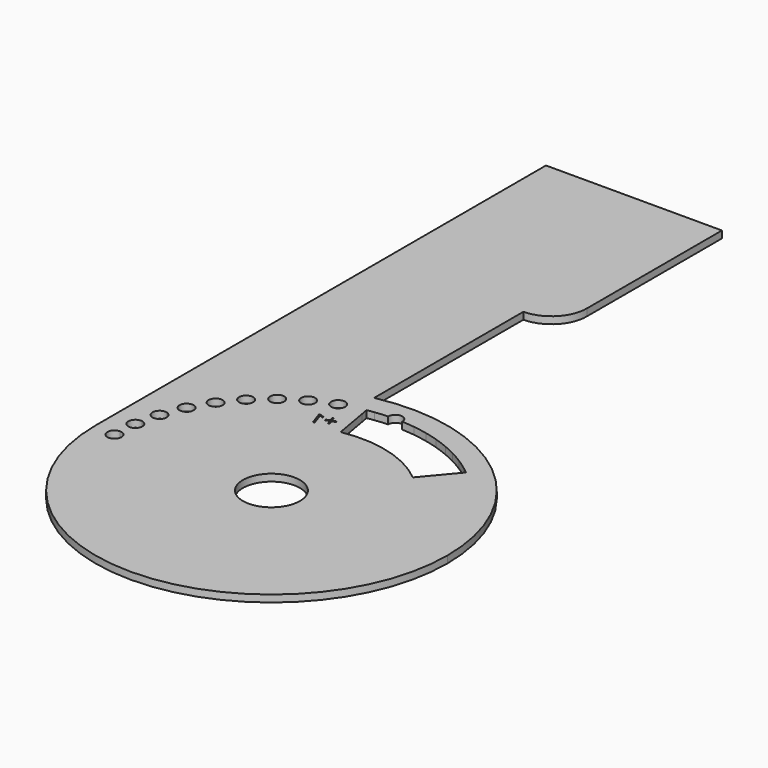
from build123d import *

# Parameters (mm, degrees)
F1_DEPTH     = 1
F7_DEPTH     = 1
F8_TEXT_SIZE = 2.7777777778
F9_DEPTH     = 1
F10_DEPTH    = 1
F13_DEPTH    = 1


# Not quite as in the source:
# - Text() gives the source's letters only with a copy of the font that has no kerning and outlines rounded to 1/6400 em; it was checked with that copy


with BuildPart() as f1:
    # F0 (on Top) → F1 (new body)
    with BuildSketch(Plane.XY):
        with BuildLine():
            ThreePointArc((-25, 0), (0, 25), (25, 0))
            Line((25, 0), (25, 35))
            Line((25, 35), (0, 60))
            Line((0, 60), (0, 65))
            Line((0, 65), (25, 65))
            Line((25, 65), (25, 80))
            Line((25, 80), (-25, 80))
            Line((-25, 80), (-25, 0))
        make_face()
        with BuildLine():
            Line((25, 0), (4.05, 0))
            ThreePointArc((4.05, 0), (0, -4.05), (-4.05, 0))
            Line((-4.05, 0), (-25, 0))
            ThreePointArc((-25, 0), (0, -25), (25, 0))
        make_face()
        with BuildLine():
            ThreePointArc((-4.05, 0), (0, 4.05), (4.05, 0))
            Line((4.05, 0), (25, 0))
            ThreePointArc((25, 0), (0, 25), (-25, 0))
            Line((-25, 0), (-4.05, 0))
        make_face()
        Polygon((0, 60), (25, 35), (25, 65), (0, 65), align=None)
    extrude(amount=-F1_DEPTH)

    # F6 (on face) → F7 (cut, through all)
    with BuildSketch(Plane.XY):
        with BuildLine():
            ThreePointArc((-17.4292995996, 13.4245862307), (-18.0213449744, 12.6186815997), (-18.5761561652, 11.7867053125))
            ThreePointArc((-18.5761561652, 11.7867053125), (-17.5495458597, 11.7369755288), (-17.0213449744, 12.6186815997))
            ThreePointArc((-17.0213449744, 12.6186815997), (-17.1291439391, 13.0703200753), (-17.4292995996, 13.4245862307))
        make_face()
        with BuildLine():
            ThreePointArc((-17.4292995996, 13.4245862307), (-18.8404970186, 13.1922580361), (-18.5761561652, 11.7867053125))
            ThreePointArc((-18.5761561652, 11.7867053125), (-18.0213449744, 12.6186815997), (-17.4292995996, 13.4245862307))
        make_face()
        with BuildLine():
            ThreePointArc((-16.5036059173, 14.5475424634), (-15.8254756075, 15.2824841501), (-15.1146480339, 15.9858504563))
            ThreePointArc((-15.1146480339, 15.9858504563), (-16.5448154078, 15.9771425206), (-16.5036059173, 14.5475424634))
        make_face()
        with BuildLine():
            ThreePointArc((-14.8254756075, 15.2824841501), (-14.9005897838, 15.6627290886), (-15.1146480339, 15.9858504563))
            ThreePointArc((-15.1146480339, 15.9858504563), (-15.8254756075, 15.2824841501), (-16.5036059173, 14.5475424634))
            ThreePointArc((-16.5036059173, 14.5475424634), (-15.4243087531, 14.3664791529), (-14.8254756075, 15.2824841501))
        make_face()
        with BuildLine():
            ThreePointArc((-12.2399305093, 17.569981221), (-12.288062126, 17.8764882859), (-12.4278236709, 18.1534899896))
            ThreePointArc((-12.4278236709, 18.1534899896), (-13.2399305093, 17.569981221), (-14.0246821194, 16.9501708384))
            ThreePointArc((-14.0246821194, 16.9501708384), (-12.9118692423, 16.6253247729), (-12.2399305093, 17.569981221))
        make_face()
        with BuildLine():
            ThreePointArc((-14.0246821194, 16.9501708384), (-13.2399305093, 17.569981221), (-12.4278236709, 18.1534899896))
            ThreePointArc((-12.4278236709, 18.1534899896), (-13.8417455325, 18.3686167311), (-14.0246821194, 16.9501708384))
        make_face()
        with BuildLine():
            ThreePointArc((-11.2004241025, 18.9354297528), (-10.3283743813, 19.4248470429), (-9.4349850436, 19.8741303515))
            ThreePointArc((-9.4349850436, 19.8741303515), (-10.7978459441, 20.3077946358), (-11.2004241025, 18.9354297528))
        make_face()
        with BuildLine():
            ThreePointArc((-9.3283743813, 19.4248470429), (-9.3553920234, 19.6557265161), (-9.4349850436, 19.8741303515))
            ThreePointArc((-9.4349850436, 19.8741303515), (-10.3283743813, 19.4248470429), (-11.2004241025, 18.9354297528))
            ThreePointArc((-11.2004241025, 18.9354297528), (-10.0754413083, 18.457363265), (-9.3283743813, 19.4248470429))
        make_face()
        with BuildLine():
            ThreePointArc((-8.100374472, 20.4544355437), (-7.1624993981, 20.8014086632), (-6.2098257716, 21.1054036656))
            ThreePointArc((-6.2098257716, 21.1054036656), (-7.4880675525, 21.7469272388), (-8.100374472, 20.4544355437))
        make_face()
        with BuildLine():
            ThreePointArc((-6.1624993981, 20.8014086632), (-6.1744018253, 20.9552370961), (-6.2098257716, 21.1054036656))
            ThreePointArc((-6.2098257716, 21.1054036656), (-7.1624993981, 20.8014086632), (-8.100374472, 20.4544355437))
            ThreePointArc((-8.100374472, 20.4544355437), (-6.9862539357, 19.8170624147), (-6.1624993981, 20.8014086632))
        make_face()
        with BuildLine():
            ThreePointArc((-19.3147839647, 10.5327641385), (-20.6722630649, 10.0825363761), (-20.1912997976, 8.735640359))
            ThreePointArc((-20.1912997976, 8.735640359), (-19.7734690186, 9.6441652294), (-19.3147839647, 10.5327641385))
        make_face()
        with BuildLine():
            ThreePointArc((-19.3147839647, 10.5327641385), (-19.7734690186, 9.6441652294), (-20.1912997976, 8.735640359))
            ThreePointArc((-20.1912997976, 8.735640359), (-19.2339464422, 8.8021940959), (-18.7734690186, 9.6441652294))
            ThreePointArc((-18.7734690186, 9.6441652294), (-18.9194534877, 10.1644127407), (-19.3147839647, 10.5327641385))
        make_face()
        with BuildLine():
            ThreePointArc((-20.7246742464, 7.381590437), (-21.0387046312, 6.4321775039), (-21.3092666179, 5.4694749479))
            ThreePointArc((-21.3092666179, 5.4694749479), (-20.4347849291, 5.63513234), (-20.0387046312, 6.4321775039))
            ThreePointArc((-20.0387046312, 6.4321775039), (-20.2281398945, 7.0178265521), (-20.7246742464, 7.381590437))
        make_face()
        with BuildLine():
            ThreePointArc((-20.7246742464, 7.381590437), (-21.9950093871, 6.7245492086), (-21.3092666179, 5.4694749479))
            ThreePointArc((-21.3092666179, 5.4694749479), (-21.0387046312, 6.4321775039), (-20.7246742464, 7.381590437))
        make_face()
        with BuildLine():
            ThreePointArc((-21.624254267, 4.0486574808), (-21.7858975123, 3.0618082211), (-21.9025285727, 2.0686329114))
            ThreePointArc((-21.9025285727, 2.0686329114), (-21.1213040503, 2.3146030751), (-20.7858975123, 3.0618082211))
            ThreePointArc((-20.7858975123, 3.0618082211), (-21.0237809709, 3.709248085), (-21.624254267, 4.0486574808))
        make_face()
        with BuildLine():
            ThreePointArc((-21.624254267, 4.0486574808), (-22.7761655811, 3.2009813221), (-21.9025285727, 2.0686329114))
            ThreePointArc((-21.9025285727, 2.0686329114), (-21.7858975123, 3.0618082211), (-21.624254267, 4.0486574808))
        make_face()
        with BuildLine():
            ThreePointArc((-21.9913733807, 0.6160331407), (-21.9966492934, -0.3839529416), (-21.9564775837, -1.3831457327))
            ThreePointArc((-21.9564775837, -1.3831457327), (-21.2754795112, -1.0767113014), (-20.9966492934, -0.3839529416))
            ThreePointArc((-20.9966492934, -0.3839529416), (-21.2876796493, 0.3212860559), (-21.9913733807, 0.6160331407))
        make_face()
        with BuildLine():
            ThreePointArc((-21.9913733807, 0.6160331407), (-22.9964969886, -0.4014053481), (-21.9564775837, -1.3831457327))
            ThreePointArc((-21.9564775837, -1.3831457327), (-21.9966492934, -0.3839529416), (-21.9913733807, 0.6160331407))
        make_face()
    extrude(amount=-F7_DEPTH, mode=Mode.SUBTRACT)

    # F8 (on face) → F9 (cut, through all)
    with BuildSketch(Plane(origin=(0, 0, -1), x_dir=(1, 0, 0), z_dir=(0, 0, -1))):
        with Locations(Location((-4.2403159229, -16.5194937189), (0, 0, 161))):
            Text('+1', F8_TEXT_SIZE, font='Open Sans', text_align=(TextAlign.LEFT, TextAlign.BOTTOM))
    extrude(amount=-F9_DEPTH, mode=Mode.SUBTRACT)

    # F5 (on face) → F10 (cut, through all)
    with BuildSketch(Plane.XY):
        with BuildLine():
            Line((13.4985398034, 16.0869333055), (14.1413274131, 16.8529777486))
            ThreePointArc((14.1413274131, 16.8529777486), (13.7546525175, 17.170018466), (13.3608720283, 17.4781892267))
            ThreePointArc((13.3608720283, 17.4781892267), (13.1461875159, 16.7545065087), (13.4985398034, 16.0869333055))
        make_face()
        with BuildLine():
            Line((10.284601755, 12.2567110899), (13.4985398034, 16.0869333055))
            ThreePointArc((13.4985398034, 16.0869333055), (13.1461875159, 16.7545065087), (13.3608720283, 17.4781892267))
            ThreePointArc((13.3608720283, 17.4781892267), (12.6186815997, 18.0213449744), (11.8544380749, 18.5330056366))
            ThreePointArc((11.8544380749, 18.5330056366), (10.5, 18.1865334795), (10.1228346523, 19.5327473388))
            ThreePointArc((10.1228346523, 19.5327473388), (9.2976017583, 19.9387713148), (8.4561198683, 20.3099492065))
            ThreePointArc((8.4561198683, 20.3099492065), (7.1824230098, 19.7335450365), (6.5772200679, 20.9938128071))
            ThreePointArc((6.5772200679, 20.9938128071), (5.6940189923, 21.2503681784), (4.8008667385, 21.4697852472))
            ThreePointArc((4.8008667385, 21.4697852472), (3.646611731, 20.6809628133), (2.8317599799, 21.8169918966))
            ThreePointArc((2.8317599799, 21.8169918966), (1.9174263404, 21.916283358), (0.9997417022, 21.9772727273))
            ThreePointArc((0.9997417022, 21.9772727273), (0, 21), (-0.9997417022, 21.9772727273))
            ThreePointArc((-0.9997417022, 21.9772727273), (-1.9174263404, 21.916283358), (-2.8317599799, 21.8169918966))
            ThreePointArc((-2.8317599799, 21.8169918966), (-2.8231390713, 21.7415995554), (-2.8202599087, 21.6657705663))
            ThreePointArc((-2.8202599087, 21.6657705663), (-3.0542154656, 21.0229829566), (-3.646611731, 20.6809628133))
            Line((-3.646611731, 20.6809628133), (-2.7783708427, 15.7569240482))
            ThreePointArc((-2.7783708427, 15.7569240482), (4.1411047216, 15.4548132206), (10.284601755, 12.2567110899))
        make_face()
        with BuildLine():
            ThreePointArc((10.1228346523, 19.5327473388), (10.5, 18.1865334795), (11.8544380749, 18.5330056366))
            ThreePointArc((11.8544380749, 18.5330056366), (11, 19.0525588833), (10.1228346523, 19.5327473388))
        make_face()
        with BuildLine():
            Line((-3.8202599087, 21.6657705663), (-3.646611731, 20.6809628133))
            ThreePointArc((-3.646611731, 20.6809628133), (-3.0542154656, 21.0229829566), (-2.8202599087, 21.6657705663))
            ThreePointArc((-2.8202599087, 21.6657705663), (-2.8231390713, 21.7415995554), (-2.8317599799, 21.8169918966))
            ThreePointArc((-2.8317599799, 21.8169918966), (-3.3268692674, 21.7469984338), (-3.8202599087, 21.6657705663))
        make_face()
        with BuildLine():
            ThreePointArc((6.5772200679, 20.9938128071), (7.1824230098, 19.7335450365), (8.4561198683, 20.3099492065))
            ThreePointArc((8.4561198683, 20.3099492065), (7.5244431532, 20.6732376573), (6.5772200679, 20.9938128071))
        make_face()
        with BuildLine():
            ThreePointArc((2.8317599799, 21.8169918966), (3.646611731, 20.6809628133), (4.8008667385, 21.4697852472))
            ThreePointArc((4.8008667385, 21.4697852472), (3.8202599087, 21.6657705663), (2.8317599799, 21.8169918966))
        make_face()
        with BuildLine():
            ThreePointArc((1, 22), (-0.0113643702, 22.9999354235), (-0.9997417022, 21.9772727273))
            ThreePointArc((-0.9997417022, 21.9772727273), (0, 22), (0.9997417022, 21.9772727273))
            ThreePointArc((0.9997417022, 21.9772727273), (0.9999354235, 21.9886356298), (1, 22))
        make_face()
        with BuildLine():
            ThreePointArc((0.9997417022, 21.9772727273), (0, 22), (-0.9997417022, 21.9772727273))
            ThreePointArc((-0.9997417022, 21.9772727273), (0, 21), (0.9997417022, 21.9772727273))
        make_face()
    extrude(amount=-F10_DEPTH, mode=Mode.SUBTRACT)

    # F12 (on face) → F13 (cut, through all)
    with BuildSketch(Plane(origin=(0, 0, -1), x_dir=(1, 0, 0), z_dir=(0, 0, -1))):
        with BuildLine():
            Line((25, -80), (25, 0))
            ThreePointArc((25, 0), (15.8113883008, -19.364916731), (-5, -24.4948974278))
            Line((-5, -24.4948974278), (-5, -51))
            ThreePointArc((-5, -51), (-1.4644660941, -52.4644660941), (0, -56))
            Line((0, -56), (0, -80))
            Line((0, -80), (25, -80))
        make_face()
    extrude(amount=-F13_DEPTH, mode=Mode.SUBTRACT)


solid = f1.part
